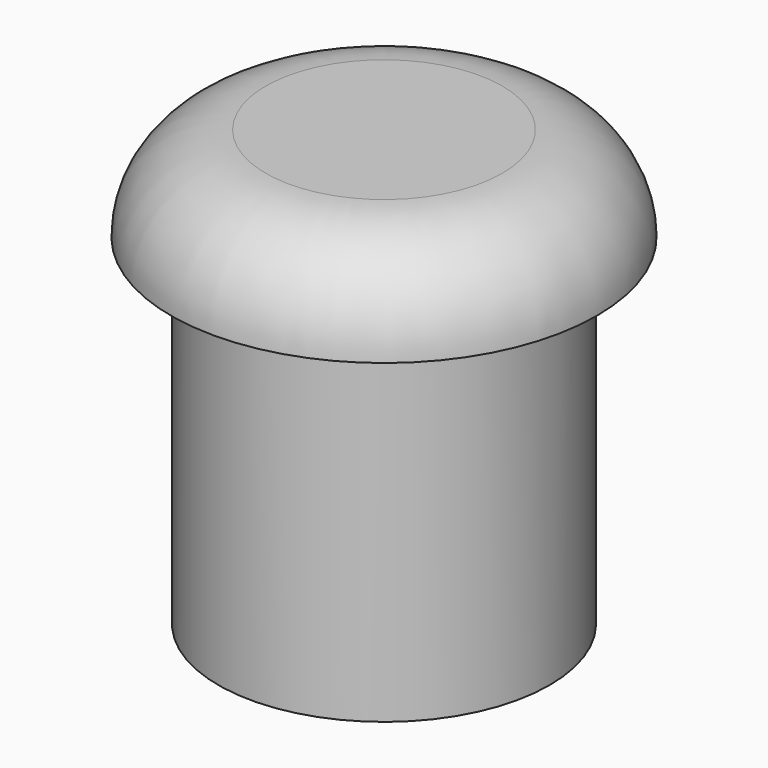
from build123d import *

# Parameters (mm, degrees)
F0_R     = 11.43
F1_DEPTH = 5.08
F2_R     = 5.07999
F3_R     = 8.89
F4_DEPTH = 18.288
F5_R     = 6.0681762548
F6_DEPTH = 12.7


# Not quite as in the source:
# - a fillet or chamfer is up to 0.001 mm smaller than in the source, because OpenCascade refuses the exact size


with BuildPart() as f1:
    # F0 (on Top) → F1 (new body)
    with BuildSketch(Plane.XY):
        Circle(F0_R)
    extrude(amount=F1_DEPTH)

    # F2 (radius 5.08 in the source; OpenCascade refuses exactly that, so slightly less here)
    f2_edges = [f1.edges().sort_by_distance(p)[0] for p in [
        (-11.43, 0, 5.08),
    ]]
    fillet(f2_edges, radius=F2_R)

    # F3 (on face) → F4 (join)
    with BuildSketch(Plane(origin=(0, 0, 0), x_dir=(1, 0, 0), z_dir=(0, 0, -1))):
        Circle(F3_R)
    extrude(amount=F4_DEPTH)

    # F5 (on face) → F6 (cut)
    with BuildSketch(Plane(origin=(0, 0, -18.288), x_dir=(1, 0, 0), z_dir=(0, 0, -1))):
        Circle(F5_R)
    extrude(amount=-F6_DEPTH, mode=Mode.SUBTRACT)


solid = f1.part
